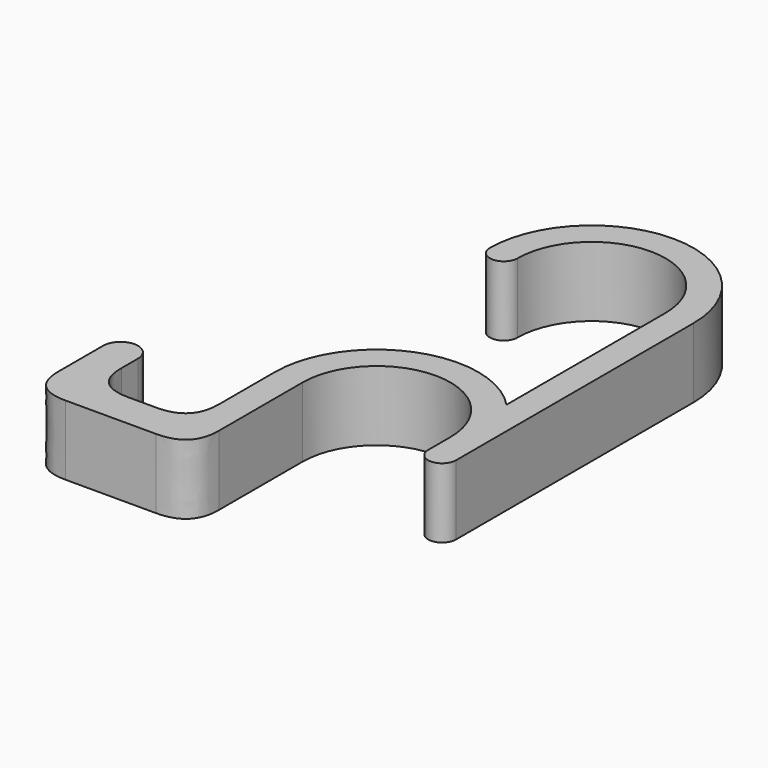
from build123d import *

# Parameters (mm, degrees)
F1_DEPTH    = 10
F2_T1_DEPTH = 10
F2_T3_DEPTH = 35


# Not quite as in the source:
# - a fillet or chamfer that OpenCascade refuses, or shapes differently, is made with other operations: its cross-section is extruded or revolved along the edge and cut away or added


with BuildPart() as f1:
    # F0 (on Top) → F1 (new body)
    with BuildSketch(Plane.XY):
        with BuildLine():
            Line((14.6, -4), (14.6, 38.55))
            ThreePointArc((14.6, 38.55), (0, 53.15), (-14.6, 38.55))
            ThreePointArc((-14.6, 38.55), (-12.6, 36.55), (-10.6, 38.55))
            ThreePointArc((-10.6, 38.55), (0, 49.15), (10.6, 38.55))
            Line((10.6, 38.55), (10.6, 10.0399203184))
            ThreePointArc((10.6, 10.0399203184), (-5.4037024344, 13.5631854665), (-14.6, 0))
            Line((-14.6, 0), (-14.6, -15))
            Line((-14.6, -15), (-28.6, -15))
            Line((-28.6, -15), (-28.6, -7))
            ThreePointArc((-28.6, -7), (-31.1, -4.5), (-33.6, -7))
            Line((-33.6, -7), (-33.6, -20))
            Line((-33.6, -20), (-10.6, -20))
            Line((-10.6, -20), (-10.6, 0))
            ThreePointArc((-10.6, 0), (0, 10.6), (10.6, 0))
            Line((10.6, 0), (10.6, -4))
            ThreePointArc((10.6, -4), (12.6, -6), (14.6, -4))
        make_face()
    extrude(amount=F1_DEPTH)

    # F2: fillet of radius 5 on 4 edges, made by hand

    # F2_s2 → F2_t1 (join)
    with BuildSketch(Plane.XY):
        with BuildLine():
            add(Edge.make_bspline(
                [(-14.6, -10), (-14.6, -15), (-19.6, -15)],
                knots=[0, 0, 0, 1, 1, 1], degree=2, weights=[1, 1, 1]))
            Line((-19.6, -15), (-14.6, -15))
            Line((-14.6, -15), (-14.6, -10))
        make_face()
        with BuildLine():
            add(Edge.make_bspline(
                [(-23.6, -15), (-28.6, -15), (-28.6, -10)],
                knots=[0, 0, 0, 1, 1, 1], degree=2, weights=[1, 1, 1]))
            Line((-28.6, -10), (-28.6, -15))
            Line((-28.6, -15), (-23.6, -15))
        make_face()
    extrude(amount=F2_T1_DEPTH)

    # F2_s4 → F2_t3 (cut)
    with BuildSketch(Plane.XY.offset(-12.5)):
        with BuildLine():
            add(Edge.make_bspline(
                [(-33.6, -15), (-33.6, -20), (-28.6, -20)],
                knots=[0, 0, 0, 1, 1, 1], degree=2, weights=[1, 1, 1]))
            Line((-28.6, -20), (-33.6, -20))
            Line((-33.6, -20), (-33.6, -15))
        make_face()
        with BuildLine():
            add(Edge.make_bspline(
                [(-10.6, -15), (-10.6, -20), (-15.6, -20)],
                knots=[0, 0, 0, 1, 1, 1], degree=2, weights=[1, 1, 1]))
            Line((-15.6, -20), (-10.6, -20))
            Line((-10.6, -20), (-10.6, -15))
        make_face()
    extrude(amount=F2_T3_DEPTH, mode=Mode.SUBTRACT)


solid = f1.part
